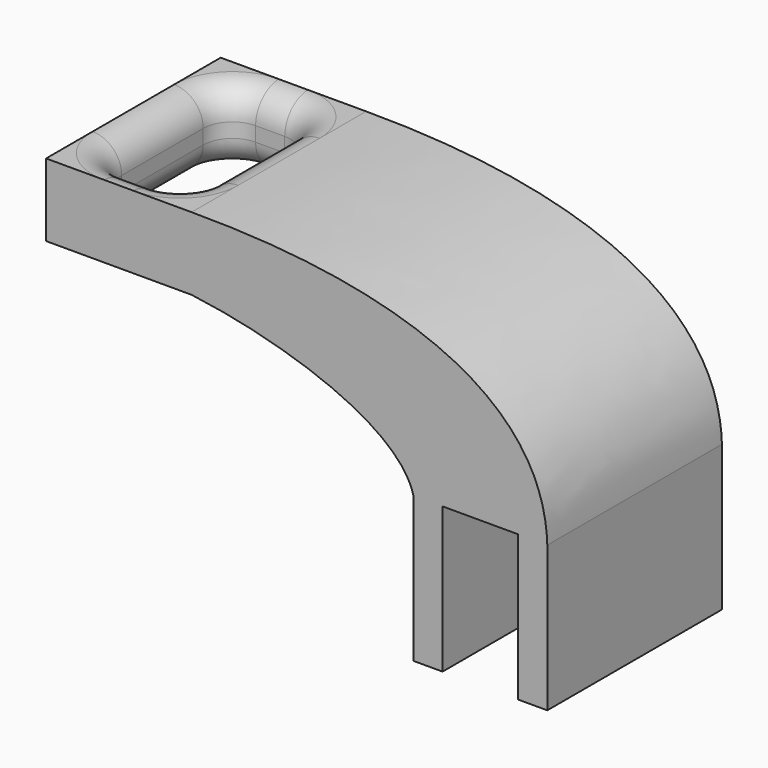
from build123d import *

# Parameters (mm, degrees)
F1_DEPTH = 19.05
F2_W     = 7.62
F2_H     = 13.97
F3_DEPTH = 6.35
F4_R     = 2.54
F5_R     = 2.53999
F6_R     = 2.53999


# Not quite as in the source:
# - a fillet or chamfer is up to 0.001 mm smaller than in the source, because OpenCascade refuses the exact size


with BuildPart() as f1:
    # F0 (on Front) → F1 (new body)
    with BuildSketch(Plane.XZ):
        with BuildLine():
            Line((-3.302, 6.35), (3.302, 6.35))
            Line((3.302, 6.35), (3.302, -6.35))
            Line((3.302, -6.35), (5.842, -6.35))
            Line((5.842, -6.35), (5.842, 6.35))
            add(Edge.make_bspline(
                [(-25.2045363516, 21.8299297452), (-6.6467649303, 21.8811389059), (5.5305822752, 17.0102007687), (5.842, 6.35)],
                knots=[0, 0, 0, 0, 34.6917229948, 34.6917229948, 34.6917229948, 34.6917229948], degree=3))
            Line((-25.2045363516, 21.8299297452), (-37.9045363516, 21.8299297452))
            Line((-37.9045363516, 21.8299297452), (-37.9045363516, 15.4799297452))
            Line((-37.9045363516, 15.4799297452), (-25.2045363516, 15.4799297452))
            add(Edge.make_bspline(
                [(-25.2045363516, 15.4799297452), (-17.7111625671, 14.5441424102), (-7.1151247248, 11.2962136045), (-5.842, 6.35)],
                knots=[0, 0, 0, 0, 21.4070883382, 21.4070883382, 21.4070883382, 21.4070883382], degree=3))
            Line((-5.842, 6.35), (-5.842, -6.35))
            Line((-5.842, -6.35), (-3.302, -6.35))
            Line((-3.302, -6.35), (-3.302, 6.35))
        make_face()
    extrude(amount=F1_DEPTH)

    # F2 (on face) → F3 (cut)
    with BuildSketch(Plane.XY.offset(21.8299297452)):
        with Locations((-31.5545363516, -9.525)):
            Rectangle(F2_W, F2_H)
    extrude(amount=-F3_DEPTH, mode=Mode.SUBTRACT)

    # F4
    f4_edges = [f1.edges().sort_by_distance(p)[0] for p in [
        (-27.744536, -2.54, 18.65493),
        (-35.364536, -2.54, 18.65493),
        (-35.364536, -16.51, 18.65493),
        (-27.744536, -16.51, 18.65493),
    ]]
    fillet(f4_edges, radius=F4_R)

    # F5 (radius 2.54 in the source; OpenCascade refuses exactly that, so slightly less here)
    f5_edges = [f1.edges().sort_by_distance(p)[0] for p in [
        (-35.364536, -9.525, 15.47993),
        (-34.620588, -15.766051, 15.47993),
        (-31.554536, -16.51, 15.47993),
        (-28.488485, -15.766051, 15.47993),
        (-27.744536, -9.525, 15.47993),
        (-31.554536, -2.54, 15.47993),
        (-34.620588, -3.283949, 15.47993),
        (-28.488485, -3.283949, 15.47993),
    ]]
    fillet(f5_edges, radius=F5_R)

    # F6 (radius 2.54 in the source; OpenCascade refuses exactly that, so slightly less here)
    f6_edges = [f1.edges().sort_by_distance(p)[0] for p in [
        (-31.554536, -16.51, 21.82993),
        (-34.620588, -15.766051, 21.82993),
        (-28.488485, -15.766051, 21.82993),
        (-35.364536, -9.525, 21.82993),
        (-27.744536, -9.525, 21.82993),
        (-28.488485, -3.283949, 21.82993),
        (-31.554536, -2.54, 21.82993),
        (-34.620588, -3.283949, 21.82993),
    ]]
    fillet(f6_edges, radius=F6_R)


solid = f1.part
